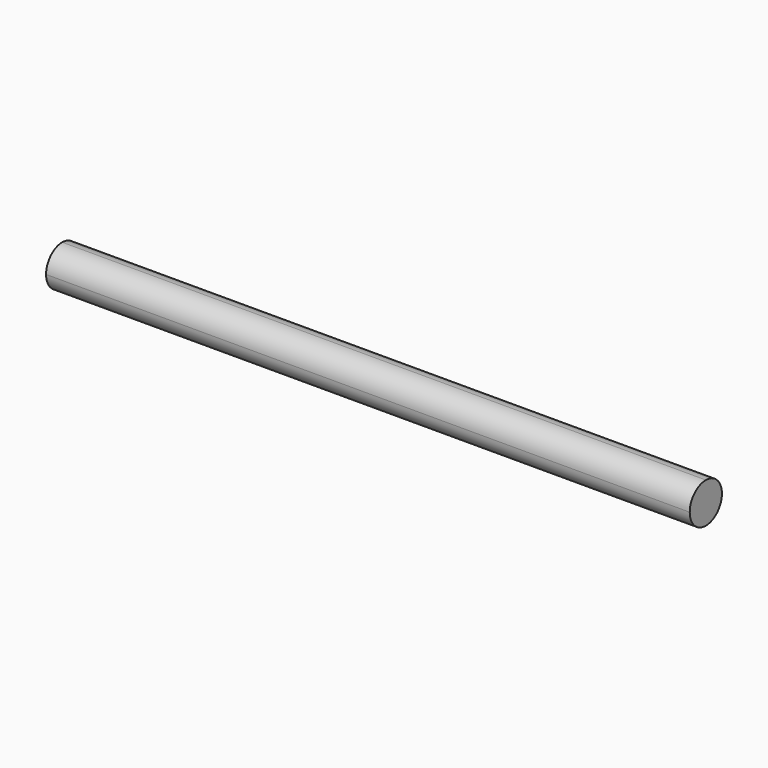
from build123d import *

# Parameters (mm, degrees)
F0_W     = 406.4
F0_H     = 25.4
F1_DEPTH = 12.7
F2_R     = 12.69999


# Not quite as in the source:
# - a fillet or chamfer is up to 0.001 mm smaller than in the source, because OpenCascade refuses the exact size


with BuildPart() as f1:
    # F0 (on Front) → F1 (new body, symmetric)
    with BuildSketch(Plane.XZ):
        with Locations((203.2, 12.7)):
            Rectangle(F0_W, F0_H)
    extrude(amount=F1_DEPTH, both=True)

    # F2 (radius 12.7 in the source; OpenCascade refuses exactly that, so slightly less here)
    f2_edges = [f1.edges().sort_by_distance(p)[0] for p in [
        (203.2, -12.7, 0),
        (203.2, -12.7, 25.4),
        (203.2, 12.7, 25.4),
        (203.2, 12.7, 0),
    ]]
    fillet(f2_edges, radius=F2_R)


solid = f1.part
